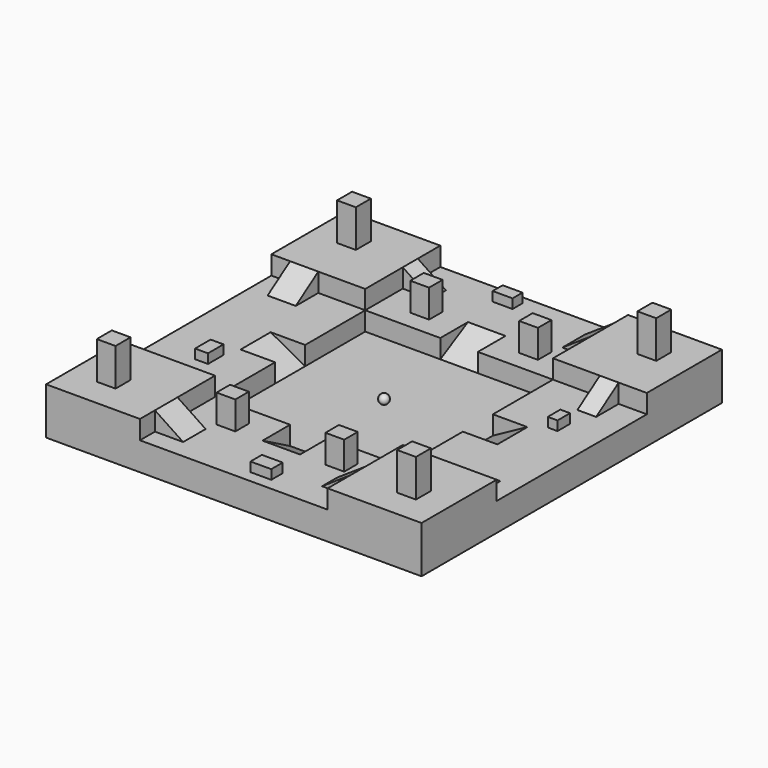
from build123d import *

# Parameters (mm, degrees)
F0_W             = 200
F0_H             = 200
F0_W_2           = 100
F0_H_2           = 100
F1_DEPTH         = 10
F2_W             = 200
F2_H             = 200
F3_DEPTH         = 5
F5_DEPTH         = 10
F5_DEPTH_BACK    = 10
F5_COPIES_COUNT  = 4
F7_W             = 50
F7_H             = 50
F8_DEPTH         = 10
F8_COPIES_COUNT  = 4
F12_DEPTH        = 10
F12_COPIES_COUNT = 4
F15_DEPTH        = 15
F15_COPIES_COUNT = 4
F9_W             = 10
F9_H             = 10
F17_DEPTH        = 20
F17_COPIES_COUNT = 4
F18_W            = 10
F18_H            = 9
F19_DEPTH        = 15
F21_W            = 5.1742345095
F21_H            = 8.3773322403
F21_W_2          = 10.5948613491
F21_H_2          = 6.6525861621
F21_W_3          = 6.898984313
F21_H_3          = 10.3484708816
F21_W_4          = 11.0876462422
F21_H_4          = 7.638156414
F22_DEPTH        = 5


# Not quite as in the source:
# - a pattern or mirror of a feature is missing from the dataset's text; its kind, count and spacing are read off the source's solid


with BuildPart() as f1:
    # F0 (on Top) → F1 (new body)
    with BuildSketch(Plane.XY):
        Rectangle(F0_W, F0_H)
        Rectangle(F0_W_2, F0_H_2, mode=Mode.SUBTRACT)
    extrude(amount=F1_DEPTH)

    # F2 (on face) → F3 (join)
    with BuildSketch(Plane(origin=(0, 0, 0), x_dir=(1, 0, 0), z_dir=(0, 0, -1))):
        Rectangle(F2_W, F2_H)
    extrude(amount=F3_DEPTH)

    # F4 (on Right) → F5 (cut, two sides)
    with BuildSketch(Plane.YZ) as f5_sk:
        Polygon((68.3940351009, 10), (50, 10), (50, 0), align=None)
    f5 = extrude(amount=-F5_DEPTH, mode=Mode.SUBTRACT) + extrude(f5_sk.sketch, amount=F5_DEPTH_BACK, mode=Mode.SUBTRACT)

    # F5_copies: F5 ×4 about axis
    f5_copies_axis = Axis((0, 0, 0), (0, 0, 1))
    for i in range(1, F5_COPIES_COUNT):
        add(f5.rotate(f5_copies_axis, i * 360 / F5_COPIES_COUNT), mode=Mode.SUBTRACT)

    # F7 (on face) → F8 (join)
    with BuildSketch(Plane.XY.offset(10)):
        with Locations((-75, 75)):
            Rectangle(F7_W, F7_H)
    f8 = extrude(amount=F8_DEPTH)

    # F8_copies: F8 ×4 about axis
    f8_copies_axis = Axis((0, 0, 0), (0, 0, 1))
    for i in range(1, F8_COPIES_COUNT):
        add(f8.rotate(f8_copies_axis, i * 360 / F8_COPIES_COUNT))

    # F11 (on line) → F12 (join)
    with BuildSketch(Plane(origin=(0, 75, 0), x_dir=(-1, 0, 0), z_dir=(0, 1, 0))):
        Polygon((50, 10), (50, 20), (35, 10), align=None)
    f12 = extrude(amount=F12_DEPTH)

    # F12_copies: F12 ×4 about axis
    f12_copies_axis = Axis((0, 0, 0), (0, 0, 1))
    for i in range(1, F12_COPIES_COUNT):
        add(f12.rotate(f12_copies_axis, i * 360 / F12_COPIES_COUNT))

    # F14 (on line) → F15 (join)
    with BuildSketch(Plane.YZ.offset(-75)):
        Polygon((50, 10), (50, 20), (35, 10), align=None)
    f15 = extrude(amount=-F15_DEPTH)

    # F15_copies: F15 ×4 about axis
    f15_copies_axis = Axis((0, 0, 0), (0, 0, 1))
    for i in range(1, F15_COPIES_COUNT):
        add(f15.rotate(f15_copies_axis, i * 360 / F15_COPIES_COUNT))

    # F9 (on face) → F17 (join)
    with BuildSketch(Plane.XY.offset(20)):
        with Locations((-80, 80)):
            Rectangle(F9_W, F9_H)
    f17 = extrude(amount=F17_DEPTH)

    # F17_copies: F17 ×4 about axis
    f17_copies_axis = Axis((0, 0, 0), (0, 0, 1))
    for i in range(1, F17_COPIES_COUNT):
        add(f17.rotate(f17_copies_axis, i * 360 / F17_COPIES_COUNT))

    # F18 (on face) → F19 (join)
    with BuildSketch(Plane.XY.offset(10)):
        with Locations((-29, 64.5)):
            Rectangle(F18_W, F18_H)
        with Locations((29, 64.5)):
            Rectangle(F18_W, F18_H)
    f19 = extrude(amount=F19_DEPTH)

    # F19_copies: F19 across plane
    add(f19.mirror(Plane(origin=(0, 0, 0), x_dir=(0, 0, -1), z_dir=(0, -1, 0))))

    # F21 (on face) → F22 (join)
    with BuildSketch(Plane.XY.offset(10)):
        with Locations((77.8486952186, 19.161650911)):
            Rectangle(F21_W, F21_H)
        with Locations((-8.1421594368, 92.4633108079)):
            Rectangle(F21_W_2, F21_H_2)
        with Locations((-74.2984488606, -23.4641870484)):
            Rectangle(F21_W_3, F21_H_3)
        with Locations((9.3516821507, -89.8668691516)):
            Rectangle(F21_W_4, F21_H_4)
    extrude(amount=F22_DEPTH)


with BuildPart() as f25:
    # F24 (on offset) → F25 (revolve)
    with BuildSketch(Plane.XY.offset(5)):
        with BuildLine():
            Line((0, 2.5), (0, -2.5))
            ThreePointArc((0, -2.5), (2.5, 0), (0, 2.5))
        make_face()
    revolve(axis=Axis((0, 0.5305833183, 5), (0, -1, 0)))


solid = Compound([f1.part, f25.part])
